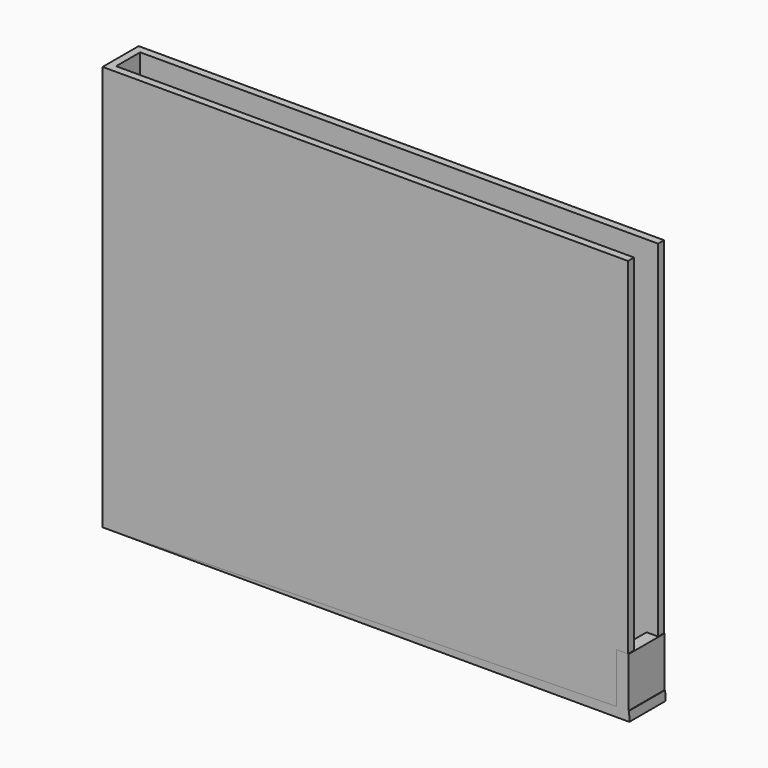
from build123d import *

# Parameters (mm, degrees)
F0_W     = 175
F0_H     = 135
F1_DEPTH = 15
F2_T     = -2.5
F4_DEPTH = 15
F5_W     = 4.0458589792
F5_H     = 19.8161639273
F6_DEPTH = 15


with BuildPart() as f1:
    # F0 (on Front) → F1 (new body)
    with BuildSketch(Plane.XZ):
        with Locations((87.5, 67.5)):
            Rectangle(F0_W, F0_H)
    extrude(amount=F1_DEPTH)

    # F2
    f2_openings = [f1.faces().sort_by_distance(p)[0] for p in [
        (87.5, -7.5, 135),
        (175, -7.5, 67.5),
    ]]
    offset(amount=F2_T, openings=f2_openings)


with BuildPart() as f4:
    # F3 (on Front) → F4 (new body)
    with BuildSketch(Plane.XZ):
        Polygon((175.3625184086, 3.230029002), (0, 0), (175.4220128059, 0), align=None)
    extrude(amount=F4_DEPTH)

    # F5 (on face) → F6 (join)
    with BuildSketch(Plane.XZ):
        with Locations((173.1846705079, 9.9080819637)):
            Rectangle(F5_W, F5_H)
    extrude(amount=F6_DEPTH)


solid = Compound([f1.part, f4.part])
